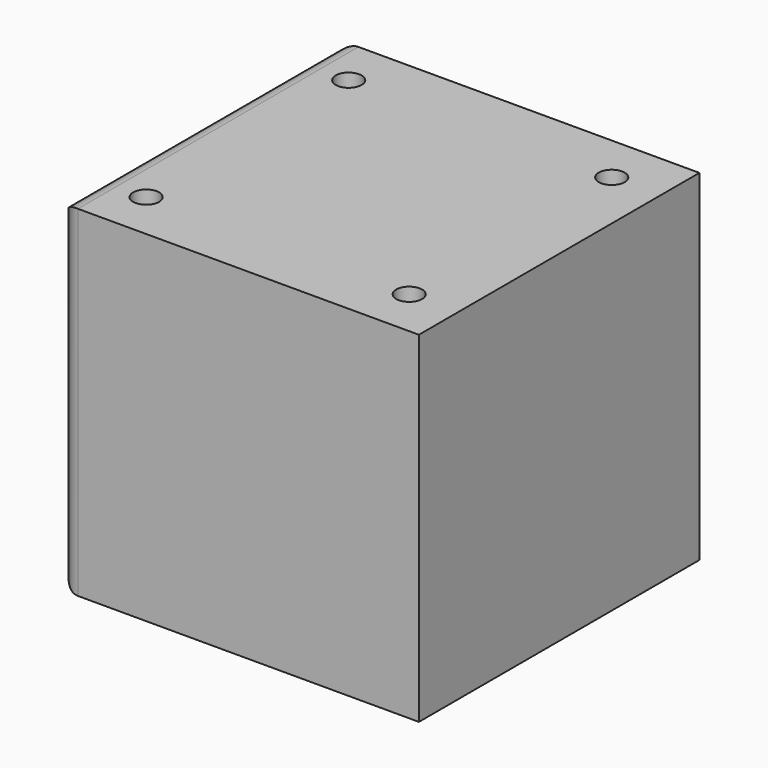
from build123d import *

# Parameters (mm, degrees)
F0_W     = 94.0087363124
F0_H     = 91.4413630962
F1_DEPTH = 88.9
F3_D     = 6.7564
F3_DEPTH = 12.7
F3_TIP   = 2.0298273432
F6_R     = 5.08


# Not quite as in the source:
# - the program builds the solid bodies; features that only make, move or delete a surface that nothing else refers to are left out


with BuildPart() as f1:
    # F0 (on Top) → F1 (new body)
    with BuildSketch(Plane.XY):
        Rectangle(F0_W, F0_H)
    extrude(amount=F1_DEPTH)

    # F3
    with Locations(Plane.XY.offset(88.9)):
        with Locations((-34.3043681562, 33.0206815481), (34.3043681562, 33.0206815481), (34.3043681562, -33.0206815481), (-34.3043681562, -33.0206815481)):
            Hole(F3_D / 2, depth=F3_DEPTH)
            with Locations((0, 0, -(F3_DEPTH + F3_TIP / 2))):  # 118° drill point
                Cone(0, F3_D / 2, F3_TIP, mode=Mode.SUBTRACT)

    # F6
    f6_edges = [f1.edges().sort_by_distance(p)[0] for p in [
        (-47.004368, 45.720682, 44.45),
        (-47.004368, -45.720682, 44.45),
        (-47.004368, 0, 0),
        (-47.004368, 0, 88.9),
    ]]
    fillet(f6_edges, radius=F6_R)


solid = f1.part
